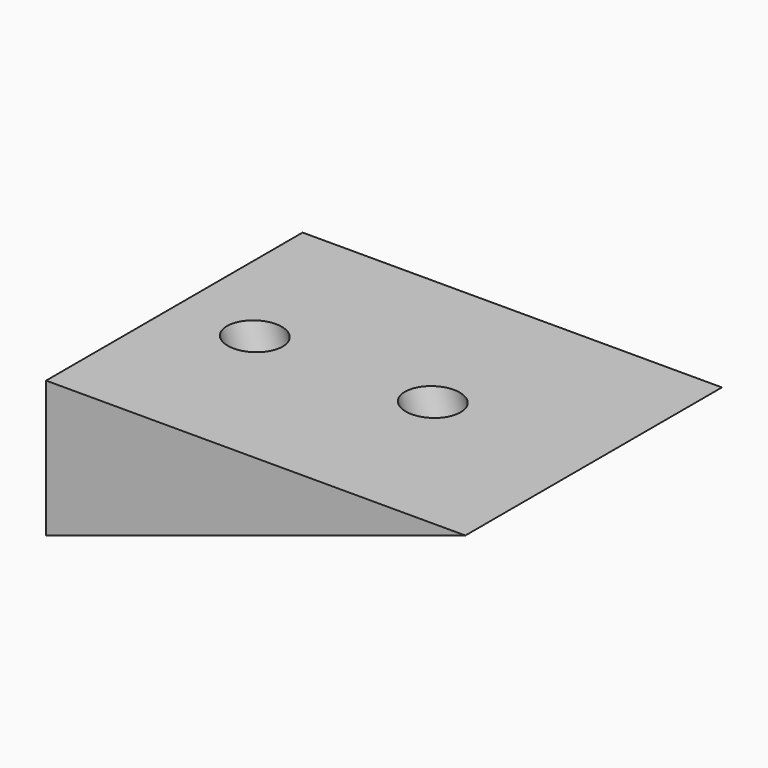
from build123d import *

# Parameters (mm, degrees)
F1_DEPTH       = 40
F3_D           = 6.6
F3_CSINK_D     = 13.44
F3_CSINK_ANGLE = 90


# Not quite as in the source:
# - a feature names something its author has since deleted; it is built from what else it names


with BuildPart() as f1:
    # F0 (on Front) → F1 (new body)
    with BuildSketch(Plane.XZ):
        Polygon((52.3067873225, 0), (0, 0), (0, -17), align=None)
    extrude(amount=F1_DEPTH)

    # F3 (through all)
    with Locations(Plane(origin=(4.997243483, 0, -15.3758677686), x_dir=(0.9510324968, 0, 0.3090909091), z_dir=(0.3090909091, 0, -0.9510324968))):
        with Locations((9.5479916781, 20), (30.6618269533, 20)):
            CounterSinkHole(F3_D / 2, F3_CSINK_D / 2, counter_sink_angle=F3_CSINK_ANGLE)


solid = f1.part
